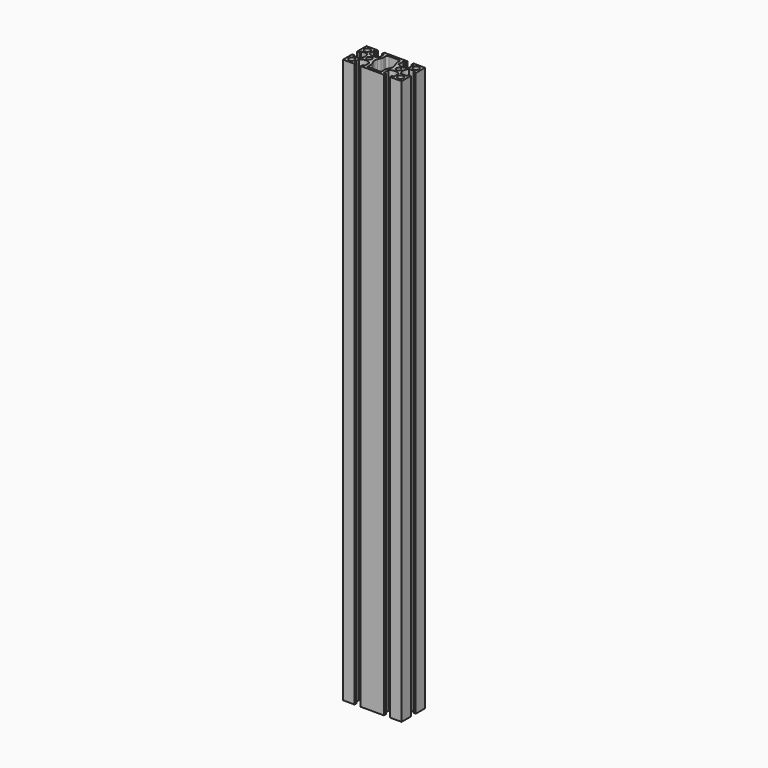
from build123d import *

# Parameters (mm, degrees)
F0_R     = 3
F0_R_2   = 2.5
F1_DEPTH = 578
F2_R     = 2
F3_R     = 7


# Not quite as in the source:
# - a feature names something its author has since deleted; it is built from what else it names


with BuildPart() as f1:
    # F0 (on Top) → F1 (new body)
    with BuildSketch(Plane.XY):
        with BuildLine():
            Line((18.15, -15), (30, -15))
            Line((30, -15), (30, -3.15))
            Line((30, -3.15), (27.5, -3.15))
            Line((27.5, -3.15), (27.5, -5.15))
            Line((27.5, -5.15), (21.5477069044, -5.15))
            ThreePointArc((21.5477069044, -5.15), (19.5, 0), (21.5477069044, 5.15))
            Line((21.5477069044, 5.15), (27.5, 5.15))
            Line((27.5, 5.15), (27.5, 3.15))
            Line((27.5, 3.15), (30, 3.15))
            Line((30, 3.15), (30, 15))
            Line((30, 15), (18.15, 15))
            Line((18.15, 15), (18.15, 12.5))
            Line((18.15, 12.5), (20.15, 12.5))
            Line((20.15, 12.5), (20.15, 6.5477069044))
            ThreePointArc((20.15, 6.5477069044), (15, 4.5), (9.85, 6.5477069044))
            Line((9.85, 6.5477069044), (9.85, 12.5))
            Line((9.85, 12.5), (11.85, 12.5))
            Line((11.85, 12.5), (11.85, 15))
            Line((11.85, 15), (-11.85, 15))
            Line((-11.85, 15), (-11.85, 12.5))
            Line((-11.85, 12.5), (-9.85, 12.5))
            Line((-9.85, 12.5), (-9.85, 6.5477069044))
            ThreePointArc((-9.85, 6.5477069044), (-15, 4.5), (-20.15, 6.5477069044))
            Line((-20.15, 6.5477069044), (-20.15, 12.5))
            Line((-20.15, 12.5), (-18.15, 12.5))
            Line((-18.15, 12.5), (-18.15, 15))
            Line((-18.15, 15), (-30, 15))
            Line((-30, 15), (-30, 3.15))
            Line((-30, 3.15), (-27.5, 3.15))
            Line((-27.5, 3.15), (-27.5, 5.15))
            Line((-27.5, 5.15), (-21.5477069044, 5.15))
            ThreePointArc((-21.5477069044, 5.15), (-19.5, 0), (-21.5477069044, -5.15))
            Line((-21.5477069044, -5.15), (-27.5, -5.15))
            Line((-27.5, -5.15), (-27.5, -3.15))
            Line((-27.5, -3.15), (-30, -3.15))
            Line((-30, -3.15), (-30, -15))
            Line((-30, -15), (-18.15, -15))
            Line((-18.15, -15), (-18.15, -12.5))
            Line((-18.15, -12.5), (-20.15, -12.5))
            Line((-20.15, -12.5), (-20.15, -6.5477069044))
            ThreePointArc((-20.15, -6.5477069044), (-15, -4.5), (-9.85, -6.5477069044))
            Line((-9.85, -6.5477069044), (-9.85, -12.5))
            Line((-9.85, -12.5), (-11.85, -12.5))
            Line((-11.85, -12.5), (-11.85, -15))
            Line((-11.85, -15), (11.85, -15))
            Line((11.85, -15), (11.85, -12.5))
            Line((11.85, -12.5), (9.85, -12.5))
            Line((9.85, -12.5), (9.85, -6.5477069044))
            ThreePointArc((9.85, -6.5477069044), (15, -4.5), (20.15, -6.5477069044))
            Line((20.15, -6.5477069044), (20.15, -12.5))
            Line((20.15, -12.5), (18.15, -12.5))
            Line((18.15, -12.5), (18.15, -15))
        make_face()
        with Locations((-25, -10)):
            Circle(F0_R, mode=Mode.SUBTRACT)
        with Locations((25, -10)):
            Circle(F0_R, mode=Mode.SUBTRACT)
        with Locations((-15, 0)):
            Circle(F0_R_2, mode=Mode.SUBTRACT)
        with Locations((-25, 10)):
            Circle(F0_R, mode=Mode.SUBTRACT)
        Polygon((-7, 7), (-7, 12.5), (0, 12.5), (7, 12.5), (7, 7), (10, 0), (7, -7), (7, -12.5), (0, -12.5), (-7, -12.5), (-7, -7), (-10, 0), align=None, mode=Mode.SUBTRACT)
        with Locations((15, 0)):
            Circle(F0_R_2, mode=Mode.SUBTRACT)
        with Locations((25, 10)):
            Circle(F0_R, mode=Mode.SUBTRACT)
    extrude(amount=F1_DEPTH)

    # F2
    f2_edges = [f1.edges().sort_by_distance(p)[0] for p in [
        (-7, 12.5, 289),
        (7, 12.5, 289),
    ]]
    fillet(f2_edges, radius=F2_R)

    # F3
    f3_edges = [f1.edges().sort_by_distance(p)[0] for p in [
        (-7, 7, 289),
        (-10, 0, 289),
        (7, 7, 289),
        (10, 0, 289),
    ]]
    fillet(f3_edges, radius=F3_R)


solid = f1.part
